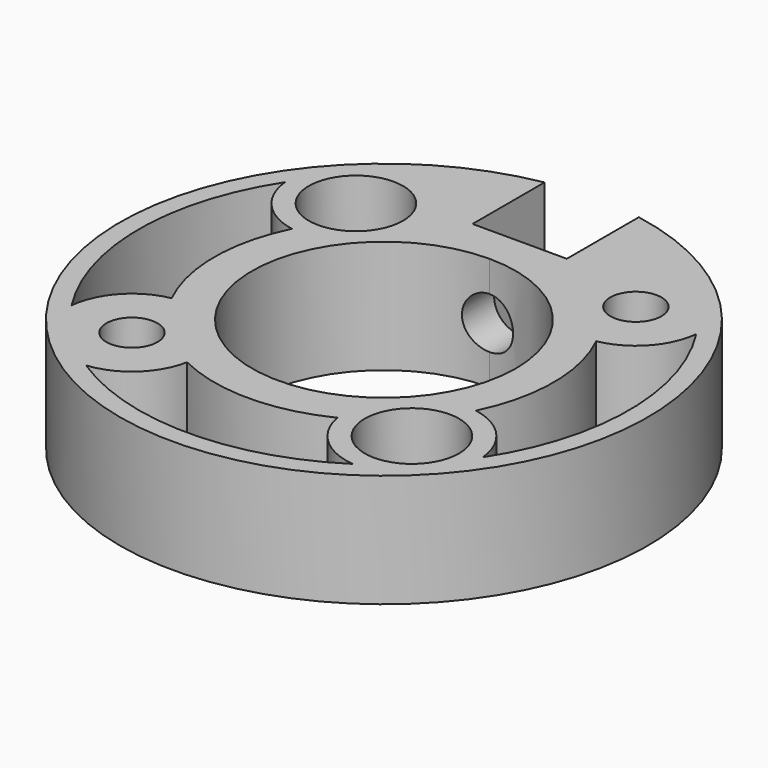
from build123d import *

# Parameters (mm, degrees)
F0_R             = 2.15265
F1_DEPTH         = 9.525
F2_R             = 2.15265
F3_REACH         = 42.6021136501
F6_R             = 3.96875
F7_DEPTH         = 6.35
F8_R             = 3.96875
F9_DEPTH         = 6.35
F11_DEPTH        = 9.525
F11_COPIES_COUNT = 3
F11_COPIES_ANGLE = 180


# Not quite as in the source:
# - a pattern or mirror of a feature is missing from the dataset's text; its kind, count and spacing are read off the source's solid


with BuildPart() as f1:
    # F0 (on Top) → F1 (new body)
    with BuildSketch(Plane.XY):
        with BuildLine():
            Line((3.96875, 14.2875), (0, 14.2875))
            Line((0, 14.2875), (-3.96875, 14.2875))
            Line((-3.96875, 14.2875), (-3.96875, 21.8677764859))
            ThreePointArc((-3.96875, 21.8677764859), (0, -22.225), (3.96875, 21.8677764859))
            Line((3.96875, 21.8677764859), (3.96875, 14.2875))
        make_face()
        with Locations((-11.7865861589, -11.7865861589)):
            Circle(F0_R, mode=Mode.SUBTRACT)
        with Locations((11.7865861589, -11.7865861589)):
            Circle(F0_R, mode=Mode.SUBTRACT)
        with Locations((-11.7865861589, 11.7865861589)):
            Circle(F0_R, mode=Mode.SUBTRACT)
        with BuildLine():
            ThreePointArc((0, 11.1125), (7.8577241059, 7.8577241059), (11.1125, 0))
            ThreePointArc((11.1125, 0), (-7.8577241059, -7.8577241059), (0, 11.1125))
        make_face(mode=Mode.SUBTRACT)
        with Locations((11.7865861589, 11.7865861589)):
            Circle(F0_R, mode=Mode.SUBTRACT)
    extrude(amount=F1_DEPTH)

    f3_end = f1.faces().sort_by_distance((0, -11.1125, 4.7625))[0]
    # F2 (on face) → F3 (cut, up to a face of the model that its end follows)
    with BuildSketch(Plane(origin=(0, 14.2875, 0), x_dir=(-1, 0, 0), z_dir=(0, 1, 0))):
        with Locations((0, 4.7625)):
            Circle(F2_R)
    f3_long = extrude(amount=-F3_REACH, mode=Mode.PRIVATE)
    add(split(f3_long, bisect_by=f3_end, keep=Keep.ALL, mode=Mode.PRIVATE).solids().sort_by_distance((0, 14.2875, 4.7625))[0], mode=Mode.SUBTRACT)

    # F6 (on face) → F7 (cut, through all)
    with BuildSketch(Plane.XY.offset(9.525)):
        with Locations((-11.7865861589, 11.7865861589)):
            Circle(F6_R)
        with Locations((11.7865861589, -11.7865861589)):
            Circle(F6_R)
    extrude(amount=-F7_DEPTH, mode=Mode.SUBTRACT)

    # F8 (on face) → F9 (cut, through all)
    with BuildSketch(Plane(origin=(0, 0, 0), x_dir=(1, 0, 0), z_dir=(0, 0, -1))):
        with Locations((11.7865861589, -11.7865861589)):
            Circle(F8_R)
        with Locations((-11.7865861589, 11.7865861589)):
            Circle(F8_R)
    extrude(amount=-F9_DEPTH, mode=Mode.SUBTRACT)

    # F10 (on face) → F11 (cut, through all)
    with BuildSketch(Plane.XY.offset(9.525)):
        with BuildLine():
            ThreePointArc((-12.8109235396, -6.3255746232), (-14.2875, 0), (-12.8109235396, 6.3255746232))
            ThreePointArc((-12.8109235396, 6.3255746232), (-15.8788163052, 8.0281867), (-17.3148424047, 11.229543123))
            ThreePointArc((-17.3148424047, 11.229543123), (-20.6375, 0), (-17.3148424047, -11.229543123))
            ThreePointArc((-17.3148424047, -11.229543123), (-15.8788163052, -8.0281867), (-12.8109235396, -6.3255746232))
        make_face()
    f11 = extrude(amount=-F11_DEPTH, mode=Mode.SUBTRACT)

    # F11_copies: F11 ×3 about axis
    f11_copies_axis = Axis((0, 0, 0), (0, 0, 1))
    for i in range(1, F11_COPIES_COUNT):
        add(f11.rotate(f11_copies_axis, i * F11_COPIES_ANGLE / (F11_COPIES_COUNT - 1)), mode=Mode.SUBTRACT)


solid = f1.part
